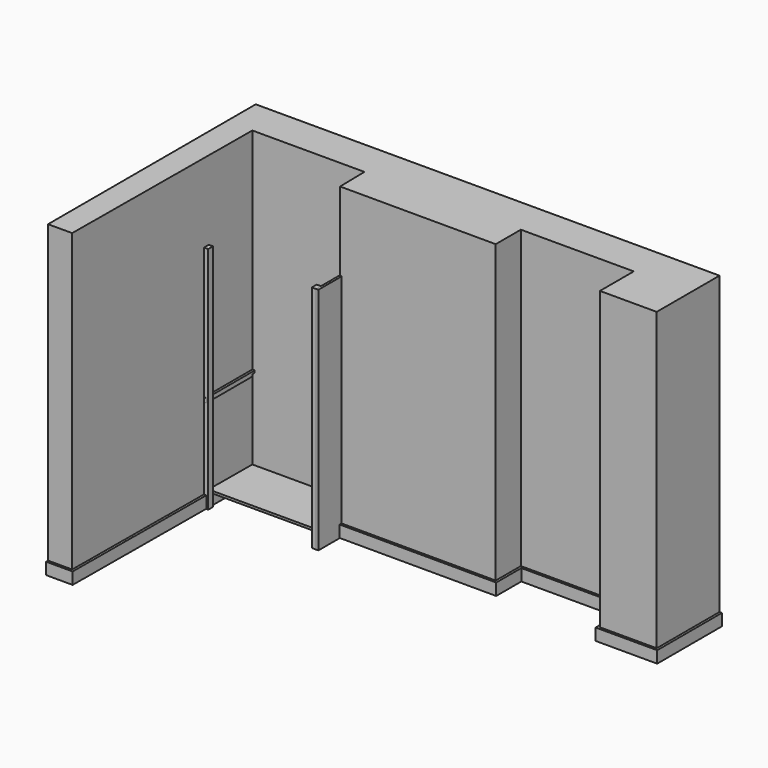
from build123d import *

# Parameters (mm, degrees)
F1_DEPTH   = 2550
F2_DEPTH   = 98
F3_W       = 35
F3_H       = 50
F4_DEPTH   = 1900
F5_OFFSET  = 2
F6_W       = 35
F6_H       = 50
F7_DEPTH   = 1900
F10_DEPTH  = 19
F11_W      = 20
F11_H      = 35
F12_DEPTH  = 500
F13_OFFSET = 1
F14_W      = 21
F14_H      = 17.5
F15_DEPTH  = 20
F17_DEPTH  = 19


# Not quite as in the source:
# - a feature names something its author has since deleted; it is built from what else it names


with BuildPart() as f1:
    # F0 (on Top) → F1 (new body)
    with BuildSketch(Plane.XY):
        Polygon((-211.8216594828, -1849.9622289028), (-11.8216594828, -1849.9622289028), (0, 0), (928, 0), (933.3707714659, -257.944092419), (2223.3691331874, -260), (2223.3691331874, 0), (3158.3691331874, 0), (3158.3691331874, -350), (3628.3691331874, -350), (3628.3691331874, 300), (-211.8216594828, 300), align=None)
    extrude(amount=F1_DEPTH)

    # F0 (on Top) → F2 (join)
    with BuildSketch(Plane.XY):
        Polygon((0, 0), (-11.8216594828, -1849.9622289028), (-211.8216594828, -1849.9622289028), (-211.8216594828, -1869.9622289028), (8.0509445283, -1869.9622289028), (19.872604011, -20), (908.4120942515, -20), (913.7822162245, -277.9128989735), (2243.3691331874, -280.0318999763), (2243.3691331874, -20), (3138.3691331874, -20), (3138.3691331874, -370), (3648.3691331874, -370), (3648.3691331874, 300), (3628.3691331874, 300), (3628.3691331874, -350), (3158.3691331874, -350), (3158.3691331874, 0), (2223.3691331874, 0), (2223.3691331874, -260), (933.3707714659, -257.944092419), (928, 0), align=None)
    extrude(amount=F2_DEPTH)


with BuildPart() as f4:
    # F3 (on Top) → F4 (new body)
    with BuildSketch(Plane.XY):
        with Locations((17.5, -475)):
            Rectangle(F3_W, F3_H)
    extrude(amount=F4_DEPTH)

    # F5: cut F1, made larger all round first
    f5_tool = offset(f1.part, amount=F5_OFFSET, kind=Kind.INTERSECTION, mode=Mode.PRIVATE)
    add(f5_tool, mode=Mode.SUBTRACT)


with BuildPart() as f7:
    # F6 (on Top) → F7 (new body, through all)
    with BuildSketch(Plane.XY):
        with Locations((910.5, -475)):
            Rectangle(F6_W, F6_H)
    extrude(amount=F7_DEPTH)


with BuildPart() as f10:
    # F9 (on face) → F10 (new body)
    with BuildSketch(Plane.XY.offset(98)):
        Polygon((1.9872604011, -2), (-0.888278392, -451.9908124358), (926.0412094252, -451.9908124358), (926.0412094252, -2), align=None)
    extrude(amount=F10_DEPTH)


with BuildPart() as f12:
    # F11 (on face) → F12 (new body, through all)
    with BuildSketch(Plane.XZ.offset(500)):
        with Locations((10, 790.5)):
            Rectangle(F11_W, F11_H)
    extrude(amount=-F12_DEPTH)


with BuildPart() as f4_1:
    add(f4.part)

    # F13: cut F12, made larger all round first
    f13_tool = offset(f12.part, amount=F13_OFFSET, kind=Kind.INTERSECTION, mode=Mode.PRIVATE)
    add(f13_tool, mode=Mode.SUBTRACT)


with BuildPart() as f12_1:
    add(f12.part)

    # F14 (on face) → F15 (cut, through all)
    with BuildSketch(Plane.YZ.offset(20)):
        with Locations((-10.5, 781.75)):
            Rectangle(F14_W, F14_H)
    extrude(amount=-F15_DEPTH, mode=Mode.SUBTRACT)


with BuildPart() as f17:
    # F16 (on face) → F17 (new body)
    with BuildSketch(Plane.YZ.offset(928)):
        Polygon((-500, 1900), (-500, 0), (-279.9128989735, 0), (-279.9128989735, 100), (-258.944092419, 100), (-258.944092419, 1900), align=None)
    extrude(amount=F17_DEPTH)


solid = Compound([f1.part, f7.part, f10.part, f4_1.part, f12_1.part, f17.part])
